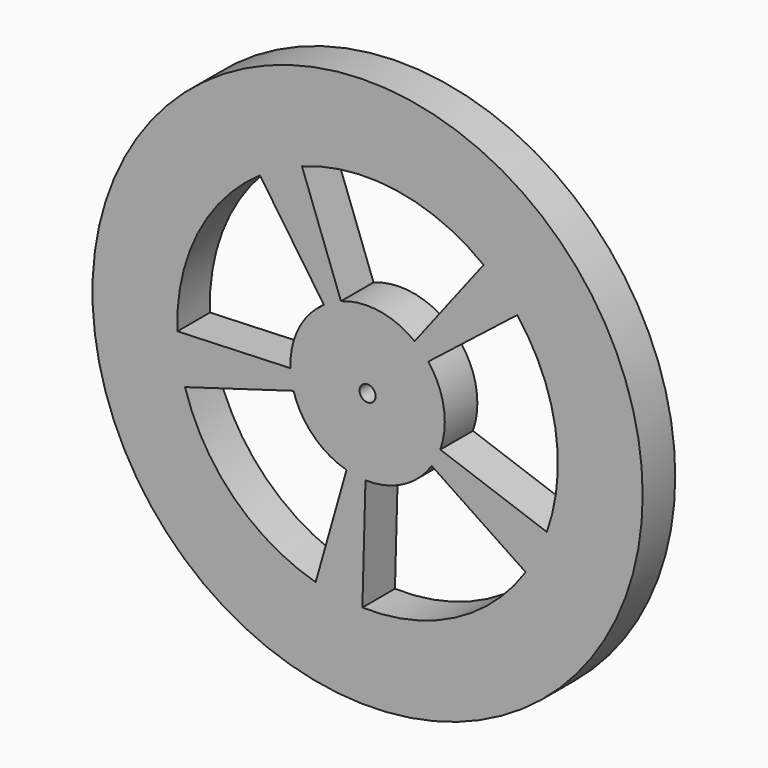
from build123d import *

# Parameters (mm, degrees)
F0_R     = 32.6
F1_DEPTH = 4.826
F2_R     = 2.45
F3_DEPTH = 25
F4_R     = 4.5746249326
F5_DEPTH = 4.826
F6_R     = 0.95
F7_DEPTH = 6.7


# Not quite as in the source:
# - a feature names something its author has since deleted; it is built from what else it names


with BuildPart() as f1:
    # F0 (on Front) → F1 (new body)
    with BuildSketch(Plane.XZ):
        Circle(F0_R)
        with BuildLine():
            ThreePointArc((-6.1511106358, -21.6948458844), (-15.8606587348, -16.0294106098), (-21.6285333971, -6.3803638683))
            Line((-21.6285333971, -6.3803638683), (-8.7761011345, -2.5889281328))
            ThreePointArc((-8.7761011345, -2.5889281328), (-6.435699664, -6.5041732629), (-2.4959052026, -8.8030084187))
            Line((-2.4959052026, -8.8030084187), (-6.1511106358, -21.6948458844))
        make_face(mode=Mode.SUBTRACT)
        with BuildLine():
            ThreePointArc((18.7322268276, -12.5541299212), (10.3436623217, -20.0377431307), (-0.6154977498, -22.5415984908))
            Line((-0.6154977498, -22.5415984908), (-0.249747424, -9.1465909619))
            ThreePointArc((-0.249747424, -9.1465909619), (4.197095798, -8.130614175), (7.6008813957, -5.09402611))
            Line((7.6008813957, -5.09402611), (18.7322268276, -12.5541299212))
        make_face(mode=Mode.SUBTRACT)
        with BuildLine():
            Line((-12.7516710164, 18.5983167596), (-5.1741813659, 7.5465453814))
            ThreePointArc((-5.1741813659, 7.5465453814), (-8.1745769317, 4.1108140298), (-9.1434356436, -0.3465322961))
            Line((-9.1434356436, -0.3465322961), (-22.5338222691, -0.854022216))
            ThreePointArc((-22.5338222691, -0.854022216), (-20.1460885038, 10.1310225543), (-12.7516710164, 18.5983167596))
        make_face(mode=Mode.SUBTRACT)
        with BuildLine():
            ThreePointArc((17.7282635002, 13.9359668938), (22.2533936178, 3.6454042971), (21.2481348677, -7.5511101598))
            Line((21.2481348677, -7.5511101598), (8.6217487379, -3.0639759628))
            ThreePointArc((8.6217487379, -3.0639759628), (9.0296475212, 1.4791773534), (7.1935082495, 5.6547271432))
            Line((7.1935082495, 5.6547271432), (17.7282635002, 13.9359668938))
        make_face(mode=Mode.SUBTRACT)
        with BuildLine():
            Line((-3.1550487991, 8.5888396815), (-7.7755574229, 21.1670311277))
            ThreePointArc((-7.7755574229, 21.1670311277), (3.4096912991, 22.2907268891), (13.7475672956, 17.8747557593))
            Line((13.7475672956, 17.8747557593), (5.5782811865, 7.2529496762))
            ThreePointArc((5.5782811865, 7.2529496762), (1.3835332766, 9.0447960548), (-3.1550487991, 8.5888396815))
        make_face(mode=Mode.SUBTRACT)
    extrude(amount=F1_DEPTH)

    # F2 (on Front) → F3 (cut, symmetric)
    with BuildSketch(Plane.XZ):
        Circle(F2_R)
    extrude(amount=F3_DEPTH, both=True, mode=Mode.SUBTRACT)

    # F4 (on Front) → F5 (join)
    with BuildSketch(Plane.XZ):
        Circle(F4_R)
    extrude(amount=F5_DEPTH)

    # F6 (on face) → F7 (cut)
    with BuildSketch(Plane(origin=(0, 0, 0), x_dir=(-1, 0, 0), z_dir=(0, 1, 0))):
        Circle(F6_R)
    extrude(amount=-F7_DEPTH, mode=Mode.SUBTRACT)


solid = f1.part
